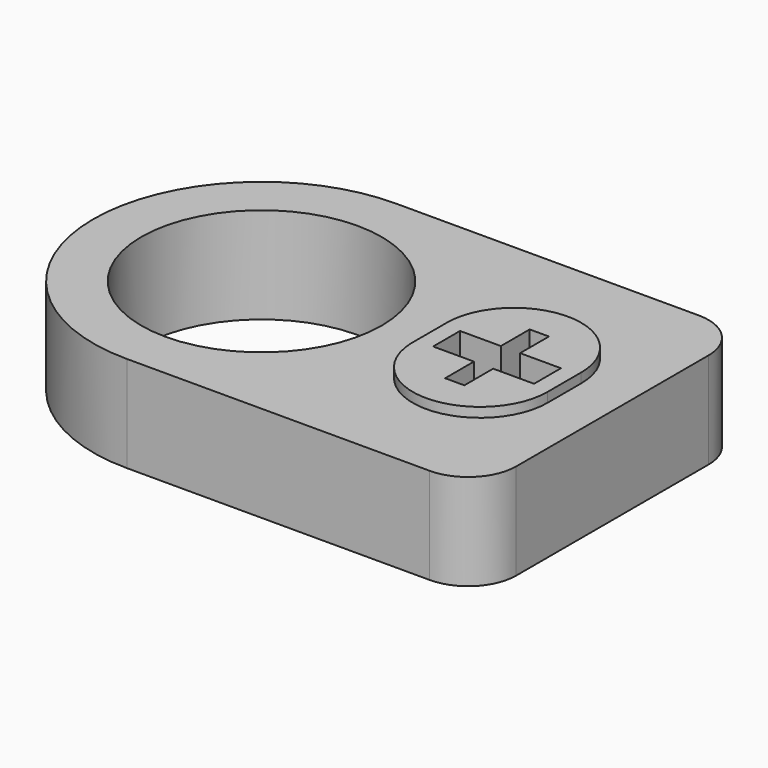
from build123d import *

# Parameters (mm, degrees)
F0_R         = 12.5
F1_DEPTH     = 10
F3_DEPTH     = 1
F4_DEPTH     = 9
F5_TEXT_SIZE = 5.5555555556
F6_DEPTH     = 1


# Not quite as in the source:
# - Text() gives the source's letters only with a copy of the font that has no kerning and outlines rounded to 1/6400 em; it was checked with that copy


with BuildPart() as f1:
    # F0 (on Top) → F1 (new body)
    with BuildSketch(Plane.XY):
        with BuildLine():
            ThreePointArc((0, 17.5), (5.1256313292, 5.1256313292), (17.5, 0))
            Line((17.5, 0), (49, 0))
            ThreePointArc((49, 0), (52.5355339059, 1.4644660941), (54, 5))
            Line((54, 5), (54, 30))
            ThreePointArc((54, 30), (52.5355339059, 33.5355339059), (49, 35))
            Line((49, 35), (17.5, 35))
            ThreePointArc((17.5, 35), (5.1256313292, 29.8743686708), (0, 17.5))
        make_face()
        with Locations((17.5, 17.5)):
            Circle(F0_R, mode=Mode.SUBTRACT)
    extrude(amount=F1_DEPTH)

    # F2 (on face) → F3 (join)
    with BuildSketch(Plane.XY.offset(10)):
        with BuildLine():
            ThreePointArc((49, 19.7), (42.1277095354, 26.6988349227), (35.0046599215, 19.9553765589))
            Line((35.0046599215, 19.9553765589), (35.0046599215, 19.4446234411))
            Line((35.0046599215, 19.4446234411), (35.0046599215, 17.5))
            Line((35.0046599215, 17.5), (35.0046599215, 15.5553765589))
            Line((35.0046599215, 15.5553765589), (35.0046599215, 15.0446234411))
            ThreePointArc((35.0046599215, 15.0446234411), (42.1277095354, 8.3011650773), (49, 15.3))
            Line((49, 15.3), (49, 17.5))
            Line((49, 17.5), (49, 19.7))
        make_face()
        Polygon((41, 23), (43, 23), (43, 19.25), (47.25, 19.25), (47.25, 15.75), (43, 15.75), (43, 12), (41, 12), (41, 15.75), (36.75, 15.75), (36.75, 19.25), (41, 19.25), align=None, mode=Mode.SUBTRACT)
    extrude(amount=F3_DEPTH)

    # F4 (cut): a face of the model
    f4_faces = [f1.faces().sort_by_distance(p)[0] for p in [
        (42, 17.5, 10),
    ]]
    extrude(f4_faces, amount=-F4_DEPTH, mode=Mode.SUBTRACT)

    # F5 (on face) → F6 (cut)
    with BuildSketch(Plane(origin=(0, 0, 0), x_dir=(1, 0, 0), z_dir=(0, 0, -1))):
        with Locations((30, -9)):
            Text('947', F5_TEXT_SIZE, font='Open Sans', text_align=(TextAlign.LEFT, TextAlign.BOTTOM))
    extrude(amount=-F6_DEPTH, mode=Mode.SUBTRACT)


solid = f1.part
